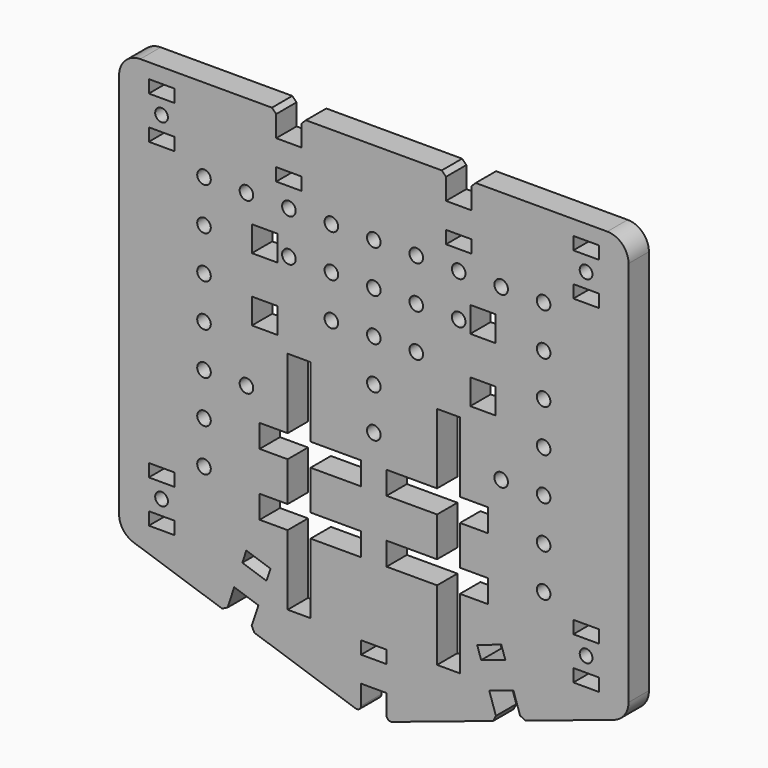
from build123d import *

# Parameters (mm, degrees)
F0_W     = 6
F0_H     = 3
F0_R     = 1.5
F0_R_2   = 1.6
F0_H_2   = 6
F1_DEPTH = 6


# Not quite as in the source:
# - ends of sketch curves that miss each other by under 0.0002 mm in the source are joined


with BuildPart() as f1:
    # F0 (on Front) → F1 (new body)
    with BuildSketch(Plane.XZ):
        with BuildLine():
            Line((24, 56.609612), (23, 55.609612))
            Line((23, 55.609612), (23, 50.609612))
            Line((23, 50.609612), (20, 50.609612))
            Line((20, 50.609612), (17, 50.609612))
            Line((17, 50.609612), (17, 55.609612))
            Line((17, 55.609612), (16, 56.609612))
            Line((16, 56.609612), (-16, 56.609612))
            Line((-16, 56.609612), (-17, 55.609612))
            Line((-17, 55.609612), (-17, 50.609612))
            Line((-17, 50.609612), (-20, 50.609612))
            Line((-20, 50.609612), (-23, 50.609612))
            Line((-23, 50.609612), (-23, 55.609612))
            Line((-23, 55.609612), (-24, 56.609612))
            Line((-24, 56.609612), (-55, 56.609612))
            ThreePointArc((-55, 56.609612), (-58.5355339059, 55.1451459059), (-60, 51.609612))
            Line((-60, 51.609612), (-60, -39.393241))
            ThreePointArc((-60, -39.393241), (-59.0562110183, -42.3167922951), (-56.5811391301, -44.1366573903))
            Line((-56.5811391301, -44.1366573903), (-35.721922, -51.08973))
            Line((-35.721922, -51.08973), (-34.457011, -50.457274))
            Line((-34.457011, -50.457274), (-32.875872, -45.713858))
            Line((-32.875872, -45.713858), (-30.029822, -46.662541))
            Line((-30.029822, -46.662541), (-27.183773, -47.611224))
            Line((-27.183773, -47.611224), (-28.764911, -52.354641))
            Line((-28.764911, -52.354641), (-28.132456, -53.619552))
            Line((-28.132456, -53.619552), (-4.316228, -61.558294))
            ThreePointArc((-4.316228, -61.558294), (-3.4152898436, -61.4208532776), (-3, -60.609611))
            Line((-3, -60.609611), (-3, -55.997037))
            Line((-3, -55.997037), (0, -55.997037))
            Line((0, -55.997037), (3, -55.997037))
            Line((3, -55.997037), (3, -60.609611))
            ThreePointArc((3, -60.609611), (3.4152894588, -61.4208530003), (4.316227166, -61.5582944981))
            Line((4.316227166, -61.5582944981), (28.132455, -53.619552))
            Line((28.132455, -53.619552), (28.764911, -52.354641))
            Line((28.764911, -52.354641), (27.183772, -47.611224))
            Line((27.183772, -47.611224), (30.029822, -46.662541))
            Line((30.029822, -46.662541), (32.875872, -45.713858))
            Line((32.875872, -45.713858), (34.45701, -50.457274))
            Line((34.45701, -50.457274), (35.721922, -51.08973))
            Line((35.721922, -51.08973), (56.581138, -44.136657))
            ThreePointArc((56.581138, -44.136657), (59.056210741, -42.3167926799), (60, -39.393241))
            Line((60, -39.393241), (60, 51.609612))
            ThreePointArc((60, 51.609612), (58.5355339059, 55.1451459059), (55, 56.609612))
            Line((55, 56.609612), (24, 56.609612))
        make_face()
        with Locations((-50, -37.997037)):
            Rectangle(F0_W, F0_H, mode=Mode.SUBTRACT)
        with Locations((-50, -32.997037)):
            Circle(F0_R, mode=Mode.SUBTRACT)
        Polygon((-25.286405, -41.919124), (-30.978505, -40.021758), (-30.029822, -37.175708), (-24.337722, -39.073075), align=None, mode=Mode.SUBTRACT)
        with Locations((-50, -27.997037)):
            Rectangle(F0_W, F0_H, mode=Mode.SUBTRACT)
        with Locations((-40, -22.997037)):
            Circle(F0_R_2, mode=Mode.SUBTRACT)
        with Locations((-40, -12.997037)):
            Circle(F0_R_2, mode=Mode.SUBTRACT)
        with Locations((-40, -2.997037)):
            Circle(F0_R_2, mode=Mode.SUBTRACT)
        Polygon((-3, -29.793713), (-14.9, -29.793713), (-14.9, -46.293713), (-20.3, -46.293713), (-20.3, -29.793713), (-26.9, -29.793713), (-26.9, -24.393713), (-20.3, -24.393713), (-20.3, -15.093713), (-26.9, -15.093713), (-26.9, -9.693713), (-20.3, -9.693713), (-20.3, 6.806287), (-14.9, 6.806287), (-14.9, -9.693713), (-3, -9.693713), (-3, -15.093713), (-14.9, -15.093713), (-14.9, -24.393713), (-3, -24.393713), align=None, mode=Mode.SUBTRACT)
        with Locations((-30, -2.997037)):
            Circle(F0_R_2, mode=Mode.SUBTRACT)
        with Locations((0, -48.497037)):
            Rectangle(F0_W, F0_H, mode=Mode.SUBTRACT)
        Polygon((30.029822, -37.175708), (30.978505, -40.021758), (25.286405, -41.919124), (24.337722, -39.073075), align=None, mode=Mode.SUBTRACT)
        with Locations((50, -37.997037)):
            Rectangle(F0_W, F0_H, mode=Mode.SUBTRACT)
        with Locations((50, -32.997037)):
            Circle(F0_R, mode=Mode.SUBTRACT)
        Polygon((14.9, -46.293713), (14.9, -29.793713), (3, -29.793713), (3, -24.393713), (14.9, -24.393713), (14.9, -15.093713), (3, -15.093713), (3, -9.693713), (14.9, -9.693713), (14.9, 6.806287), (20.3, 6.806287), (20.3, -9.693713), (26.9, -9.693713), (26.9, -15.093713), (20.3, -15.093713), (20.3, -24.393713), (26.9, -24.393713), (26.9, -29.793713), (20.3, -29.793713), (20.3, -46.293713), align=None, mode=Mode.SUBTRACT)
        with Locations((0, -2.997037)):
            Circle(F0_R_2, mode=Mode.SUBTRACT)
        with Locations((40, -22.997037)):
            Circle(F0_R_2, mode=Mode.SUBTRACT)
        with Locations((50, -27.997037)):
            Rectangle(F0_W, F0_H, mode=Mode.SUBTRACT)
        with Locations((40, -12.997037)):
            Circle(F0_R_2, mode=Mode.SUBTRACT)
        with Locations((30, -2.997037)):
            Circle(F0_R_2, mode=Mode.SUBTRACT)
        with Locations((40, -2.997037)):
            Circle(F0_R_2, mode=Mode.SUBTRACT)
        with Locations((-40, 7.002963)):
            Circle(F0_R_2, mode=Mode.SUBTRACT)
        with Locations((-40, 17.002963)):
            Circle(F0_R_2, mode=Mode.SUBTRACT)
        with Locations((-40, 27.002963)):
            Circle(F0_R_2, mode=Mode.SUBTRACT)
        with Locations((-25.720944, 12.905192)):
            Rectangle(F0_W, F0_H_2, mode=Mode.SUBTRACT)
        with Locations((-20, 27.002963)):
            Circle(F0_R_2, mode=Mode.SUBTRACT)
        with Locations((-10, 17.002963)):
            Circle(F0_R_2, mode=Mode.SUBTRACT)
        with Locations((-10, 27.002963)):
            Circle(F0_R_2, mode=Mode.SUBTRACT)
        with Locations((-50, 41.609612)):
            Rectangle(F0_W, F0_H, mode=Mode.SUBTRACT)
        with Locations((-40, 37.002963)):
            Circle(F0_R_2, mode=Mode.SUBTRACT)
        with Locations((-50, 46.609612)):
            Circle(F0_R, mode=Mode.SUBTRACT)
        with Locations((-50, 51.609612)):
            Rectangle(F0_W, F0_H, mode=Mode.SUBTRACT)
        with Locations((-25.720944, 27.905192)):
            Rectangle(F0_W, F0_H_2, mode=Mode.SUBTRACT)
        with Locations((-30, 37.002963)):
            Circle(F0_R_2, mode=Mode.SUBTRACT)
        with Locations((-20, 37.002963)):
            Circle(F0_R_2, mode=Mode.SUBTRACT)
        with Locations((-10, 37.002963)):
            Circle(F0_R_2, mode=Mode.SUBTRACT)
        with Locations((-20, 43.109612)):
            Rectangle(F0_W, F0_H, mode=Mode.SUBTRACT)
        with Locations((0, 7.002963)):
            Circle(F0_R_2, mode=Mode.SUBTRACT)
        with Locations((0, 17.002963)):
            Circle(F0_R_2, mode=Mode.SUBTRACT)
        with Locations((10, 17.002963)):
            Circle(F0_R_2, mode=Mode.SUBTRACT)
        with Locations((0, 27.002963)):
            Circle(F0_R_2, mode=Mode.SUBTRACT)
        with Locations((10, 27.002963)):
            Circle(F0_R_2, mode=Mode.SUBTRACT)
        with Locations((25.720943, 12.905192)):
            Rectangle(F0_W, F0_H_2, mode=Mode.SUBTRACT)
        with Locations((20, 27.002963)):
            Circle(F0_R_2, mode=Mode.SUBTRACT)
        with Locations((40, 7.002963)):
            Circle(F0_R_2, mode=Mode.SUBTRACT)
        with Locations((40, 17.002963)):
            Circle(F0_R_2, mode=Mode.SUBTRACT)
        with Locations((40, 27.002963)):
            Circle(F0_R_2, mode=Mode.SUBTRACT)
        with Locations((0, 37.002963)):
            Circle(F0_R_2, mode=Mode.SUBTRACT)
        with Locations((10, 37.002963)):
            Circle(F0_R_2, mode=Mode.SUBTRACT)
        with Locations((25.720943, 27.905192)):
            Rectangle(F0_W, F0_H_2, mode=Mode.SUBTRACT)
        with Locations((20, 37.002963)):
            Circle(F0_R_2, mode=Mode.SUBTRACT)
        with Locations((20, 43.109612)):
            Rectangle(F0_W, F0_H, mode=Mode.SUBTRACT)
        with Locations((30, 37.002963)):
            Circle(F0_R_2, mode=Mode.SUBTRACT)
        with Locations((40, 37.002963)):
            Circle(F0_R_2, mode=Mode.SUBTRACT)
        with Locations((50, 41.609612)):
            Rectangle(F0_W, F0_H, mode=Mode.SUBTRACT)
        with Locations((50, 46.609612)):
            Circle(F0_R, mode=Mode.SUBTRACT)
        with Locations((50, 51.609612)):
            Rectangle(F0_W, F0_H, mode=Mode.SUBTRACT)
    extrude(amount=F1_DEPTH)


solid = f1.part
